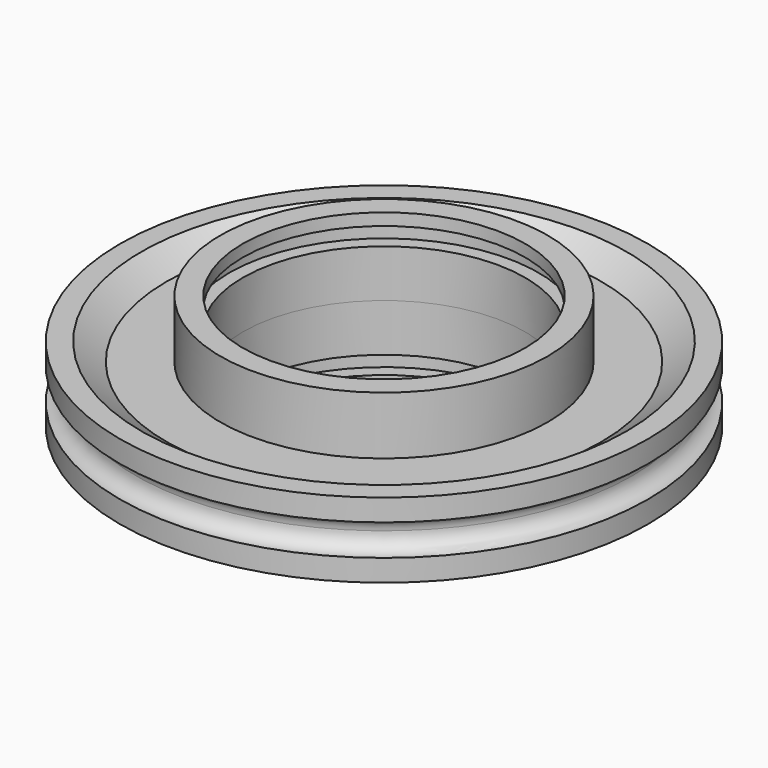
from build123d import *
from build123d import SkipClean  # not in build123d's __all__

# Parameters (mm, degrees)
F2_R = 0.889


with BuildPart() as f1:
    # F0 (on Front) → F1 (revolve)
    with BuildSketch(Plane.XZ):
        Polygon((8.0391, 2.7178), (8.0391, 0), (15.0368, 0), (15.0368, 2.1336), (13.8207983748, 2.1336), (12.3698, 1.1176), (9.3218, 1.1176), (9.3218, 4.4196), (8.0391, 4.4196), (8.0391, 3.7338), (8.8011, 3.7338), (8.8011, 2.7178), align=None)
    revolve(axis=Axis((0, 0, 19.8358264327), (0, 0, 1)))

    # F2 (on Front) → F3 (revolve, cut)
    with BuildSketch(Plane.XZ):
        with Locations((15.0368, 0)):
            Circle(F2_R)
    revolve(axis=Axis((0, 0, 19.8358264327), (0, 0, 1)), mode=Mode.SUBTRACT)

    # F4: F1 across plane


with BuildPart() as f1_1:
    add(f1.part, clean=False)
    with SkipClean():  # cleaning this boolean's faces spoils the solid; the shape is the same uncleaned
        add(f1.part.mirror(Plane.XY), clean=False)


solid = f1_1.part
